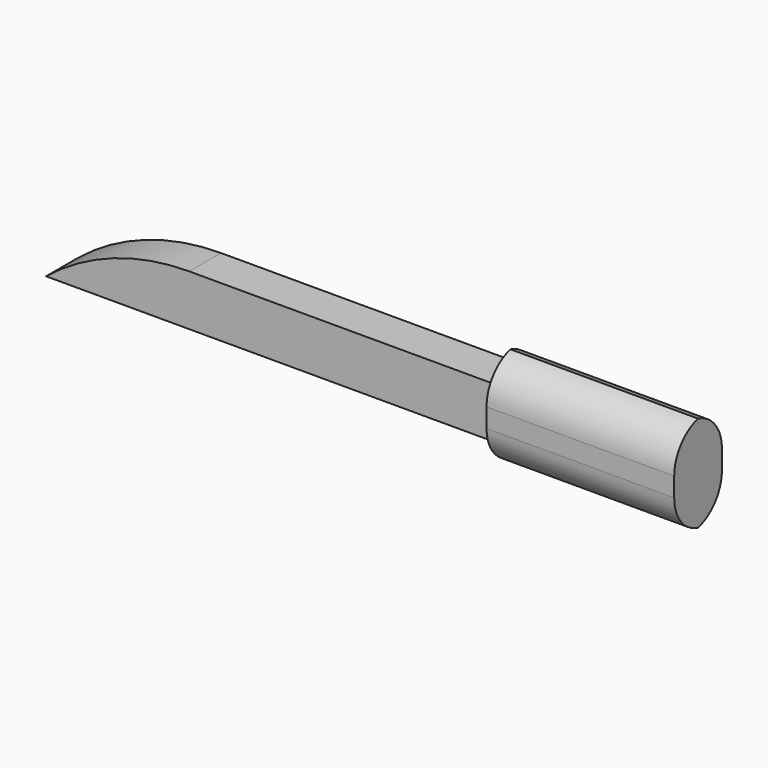
from build123d import *

# Parameters (mm, degrees)
F1_DEPTH    = 2.54
F2_DEPTH    = 3.81
F3_T1_DEPTH = 49.3776003865


# Not quite as in the source:
# - a fillet or chamfer that OpenCascade refuses, or shapes differently, is made with other operations: its cross-section is extruded or revolved along the edge and cut away or added


with BuildPart() as f1:
    # F0 (on Front) → F1 (new body, symmetric)
    with BuildSketch(Plane.XZ):
        with BuildLine():
            ThreePointArc((-36.8458546815, 12.765225481), (-46.5506501675, 11.0912601627), (-55.133856614, 6.2628253844))
            Line((-55.133856614, 6.2628253844), (2.168544932, 6.2628253844))
            Line((2.168544932, 6.2628253844), (2.168544932, 9.5140254327))
            Line((2.168544932, 9.5140254327), (2.168544932, 12.765225481))
            Line((2.168544932, 12.765225481), (-36.8458546815, 12.765225481))
        make_face()
    extrude(amount=F1_DEPTH, both=True)

    # F0 (on Front) → F2 (join, symmetric)
    with BuildSketch(Plane.XZ):
        Polygon((2.168544932, 9.5140254327), (2.168544932, 6.2628253844), (2.168544932, 3.2148253844), (26.1461453185, 3.2148253844), (26.1461453185, 9.5140254327), align=None)
        Polygon((2.168544932, 12.765225481), (2.168544932, 9.5140254327), (26.1461453185, 9.5140254327), (26.1461453185, 15.813225481), (2.168544932, 15.813225481), align=None)
    extrude(amount=F2_DEPTH, both=True)

    # F3: fillet of radius 5.08 on 4 edges, made by hand

    # F3_s2 → F3_t1 (cut)
    with BuildSketch(Plane.YZ.offset(-10.531455068)):
        with BuildLine():
            ThreePointArc((-3.81, 10.733225481), (-2.3221024484, 14.3253279294), (1.27, 15.813225481))
            Line((1.27, 15.813225481), (-3.81, 15.813225481))
            Line((-3.81, 15.813225481), (-3.81, 10.733225481))
        make_face()
        with BuildLine():
            ThreePointArc((1.27, 3.2148253844), (-2.3221024484, 4.7027229359), (-3.81, 8.2948253844))
            Line((-3.81, 8.2948253844), (-3.81, 3.2148253844))
            Line((-3.81, 3.2148253844), (1.27, 3.2148253844))
        make_face()
        with BuildLine():
            ThreePointArc((3.81, 10.733225481), (2.3221024484, 14.3253279294), (-1.27, 15.813225481))
            Line((-1.27, 15.813225481), (3.81, 15.813225481))
            Line((3.81, 15.813225481), (3.81, 10.733225481))
        make_face()
        with BuildLine():
            ThreePointArc((-1.27, 3.2148253844), (2.3221024484, 4.7027229359), (3.81, 8.2948253844))
            Line((3.81, 8.2948253844), (3.81, 3.2148253844))
            Line((3.81, 3.2148253844), (-1.27, 3.2148253844))
        make_face()
    extrude(amount=F3_T1_DEPTH, mode=Mode.SUBTRACT)


solid = f1.part
